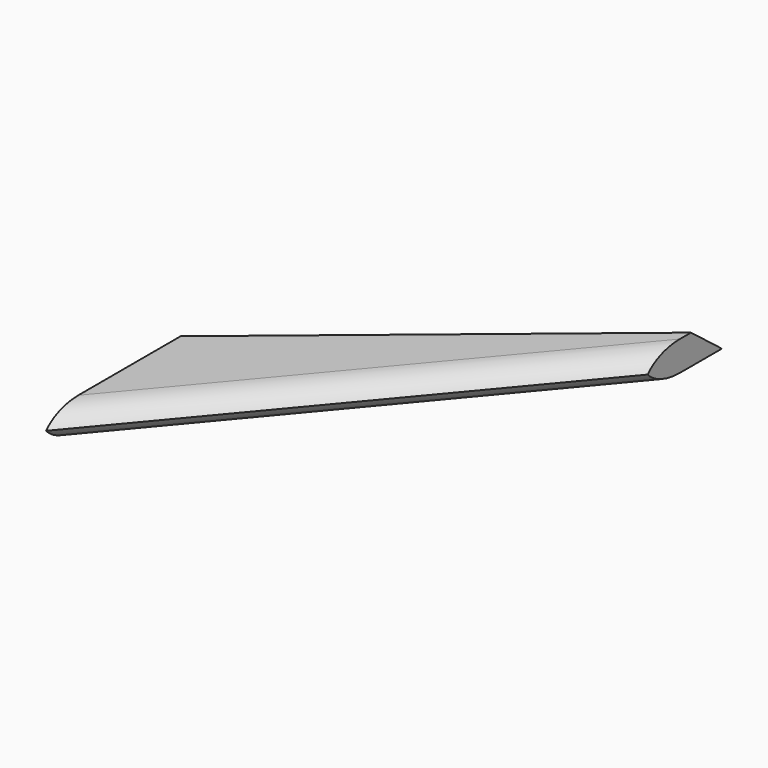
from build123d import *

# Parameters (mm, degrees)
F1_DEPTH    = 5.08
F2_T1_DEPTH = 107.0243637673
F3_SIZE     = 5.07999


# Not quite as in the source:
# - a fillet or chamfer that OpenCascade refuses, or shapes differently, is made with other operations: its cross-section is extruded or revolved along the edge and cut away or added
# - a fillet or chamfer is up to 0.001 mm smaller than in the source, because OpenCascade refuses the exact size


with BuildPart() as f1:
    # F0 (on Top) → F1 (new body)
    with BuildSketch(Plane.XY):
        Polygon((0, 36.2825095654), (0, 0), (52.3514412344, 62.6247823238), (52.3514412344, 79.496473074), align=None)
    extrude(amount=F1_DEPTH)

    # F2: fillet of radius 5.08 on 2 edges, made by hand

    # F2_s2 → F2_t1 (cut)
    with BuildSketch(Plane(origin=(-8.1454025856, -9.7438399371, 0), x_dir=(0, 0, 1), z_dir=(0.6413702823, 0.7672314911, 0))):
        with BuildLine():
            ThreePointArc((0, 0), (3.5921024484, -1.4878975516), (5.08, -5.08))
            Line((5.08, -5.08), (5.08, 0))
            Line((5.08, 0), (0, 0))
        make_face()
        with BuildLine():
            ThreePointArc((5.08, 0), (1.4878975516, -1.4878975516), (0, -5.08))
            Line((0, -5.08), (0, 0))
            Line((0, 0), (5.08, 0))
        make_face()
    extrude(amount=F2_T1_DEPTH, mode=Mode.SUBTRACT)

    # F3 (size 5.08 in the source; OpenCascade refuses exactly that, so slightly less here)
    f3_edges = [f1.edges().sort_by_distance(p)[0] for p in [
        (26.175721, 57.889491, 5.08),
    ]]
    chamfer(f3_edges, length=F3_SIZE)


solid = f1.part
